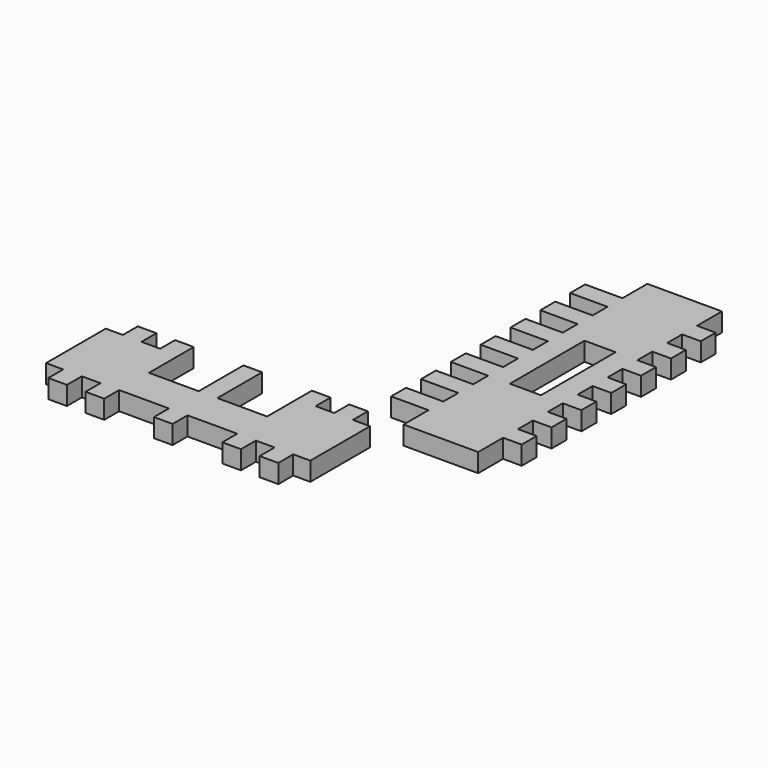
from build123d import *

# Parameters (mm, degrees)
F0_W     = 3
F0_H     = 3
F1_DEPTH = 3
F2_W     = 5
F2_H     = 15
F3_DEPTH = 25


# Not quite as in the source:
# - a feature names something its author has since deleted; it is built from what else it names


with BuildPart() as f1:
    # F0 (on Top) → F1 (new body)
    with BuildSketch(Plane.XY):
        Polygon((20.2673766234, -38.1281147589), (20.2673766234, -26.1281147589), (17.5173766234, -26.1281147589), (17.5173766234, -29.1281147589), (14.5173766234, -29.1281147589), (14.5173766234, -26.1281147589), (11.5173766234, -26.1281147589), (11.5173766234, -29.1281147589), (8.5173766234, -29.1281147589), (8.5173766234, -32.1281147589), (0.5173766234, -32.1281147589), (0.5173766234, -29.1281147589), (-2.4826233766, -29.1281147589), (-2.4826233766, -32.1281147589), (-10.4826233766, -32.1281147589), (-10.4826233766, -29.1281147589), (-13.4826233766, -29.1281147589), (-13.4826233766, -26.1281147589), (-16.4826233766, -26.1281147589), (-16.4826233766, -29.1281147589), (-19.4826233766, -29.1281147589), (-19.4826233766, -26.1281147589), (-22.2326233766, -26.1281147589), (-22.2326233766, -32.1281147589), (-22.2326233766, -38.1281147589), (-19.4826233766, -38.1281147589), (-19.4826233766, -35.1281147589), (-16.4826233766, -35.1281147589), (-16.4826233766, -38.1281147589), (-13.4826233766, -38.1281147589), (-13.4826233766, -35.1281147589), (-10.4826233766, -35.1281147589), (-10.4826233766, -38.1281147589), (-2.4826233766, -38.1281147589), (-2.4826233766, -35.1281147589), (0.5173766234, -35.1281147589), (0.5173766234, -38.1281147589), (8.5173766234, -38.1281147589), (8.5173766234, -35.1281147589), (11.5173766234, -35.1281147589), (11.5173766234, -38.1281147589), (14.5173766234, -38.1281147589), (14.5173766234, -35.1281147589), (17.5173766234, -35.1281147589), (17.5173766234, -38.1281147589), align=None)
        with Locations((16.0173766234, -27.6281147589)):
            Rectangle(F0_W, F0_H)
        with Locations((16.0173766234, -24.6281147589)):
            Rectangle(F0_W, F0_H)
        with Locations((16.0173766234, -39.6281147589)):
            Rectangle(F0_W, F0_H)
        with Locations((16.0173766234, -36.6281147589)):
            Rectangle(F0_W, F0_H)
        with Locations((10.0173766234, -27.6281147589)):
            Rectangle(F0_W, F0_H)
        with Locations((10.0173766234, -24.6281147589)):
            Rectangle(F0_W, F0_H)
        with Locations((10.0173766234, -39.6281147589)):
            Rectangle(F0_W, F0_H)
        with Locations((10.0173766234, -36.6281147589)):
            Rectangle(F0_W, F0_H)
        Polygon((0.5173766234, -27.6126158823), (0.5173766234, -26.1281147589), (-2.4826233766, -26.1281147589), (-2.4826233766, -29.1281147589), (0.5173766234, -29.1281147589), align=None)
        with Locations((-0.9826233766, -24.6281147589)):
            Rectangle(F0_W, F0_H)
        with Locations((-0.9826233766, -39.6281147589)):
            Rectangle(F0_W, F0_H)
        with Locations((-0.9826233766, -36.6281147589)):
            Rectangle(F0_W, F0_H)
        with Locations((-11.9826233766, -27.6281147589)):
            Rectangle(F0_W, F0_H)
        with Locations((-11.9826233766, -24.6281147589)):
            Rectangle(F0_W, F0_H)
        with Locations((-11.9826233766, -39.6281147589)):
            Rectangle(F0_W, F0_H)
        with Locations((-11.9826233766, -36.6281147589)):
            Rectangle(F0_W, F0_H)
        with Locations((-17.9826233766, -27.6281147589)):
            Rectangle(F0_W, F0_H)
        with Locations((-17.9826233766, -24.6281147589)):
            Rectangle(F0_W, F0_H)
        with Locations((-17.9826233766, -39.6281147589)):
            Rectangle(F0_W, F0_H)
        with Locations((-17.9826233766, -36.6281147589)):
            Rectangle(F0_W, F0_H)
    extrude(amount=F1_DEPTH)


with BuildPart() as f1b:
    # F0 (on Top) → F1, piece 2 (new body)
    with BuildSketch(Plane.XY):
        with Locations((18.7673766234, -16.6281147589)):
            Rectangle(F0_W, F0_H)
        with Locations((21.7673766234, -16.6281147589)):
            Rectangle(F0_W, F0_H)
        Polygon((23.2673766234, -15.1281147589), (23.2673766234, -18.1281147589), (23.2673766234, -23.1281147589), (35.2673766234, -23.1281147589), (35.2673766234, -18.1281147589), (35.2673766234, -15.1281147589), (35.2673766234, -12.1281147589), (35.2673766234, -9.1281147589), (35.2673766234, -6.1281147589), (35.2673766234, -3.1281147589), (35.2673766234, -0.1281147589), (35.2673766234, 2.8718852411), (35.2673766234, 5.8718852411), (35.2673766234, 8.8718852411), (35.2673766234, 11.8718852411), (35.2673766234, 14.8718852411), (35.2673766234, 17.8718852411), (35.2673766234, 20.8718852411), (35.2673766234, 25.8718852411), (29.2673766234, 25.8718852411), (23.2673766234, 25.8718852411), (23.2673766234, 20.8718852411), (23.2673766234, 17.8718852411), (23.2673766234, 14.8718852411), (23.2673766234, 11.8718852411), (23.2673766234, 8.8718852411), (23.2673766234, 5.8718852411), (23.2673766234, 2.8718852411), (23.2673766234, -0.1281147589), (23.2673766234, -3.1281147589), (23.2673766234, -6.1281147589), (23.2673766234, -9.1281147589), (23.2673766234, -12.1281147589), align=None)
        with Locations((18.7673766234, -10.6281147589)):
            Rectangle(F0_W, F0_H)
        with Locations((21.7673766234, -10.6281147589)):
            Rectangle(F0_W, F0_H)
        with Locations((18.7673766234, -4.6281147589)):
            Rectangle(F0_W, F0_H)
        with Locations((21.7673766234, -4.6281147589)):
            Rectangle(F0_W, F0_H)
        with Locations((36.7673766234, -16.6281147589)):
            Rectangle(F0_W, F0_H)
        with Locations((18.7673766234, 1.3718852411)):
            Rectangle(F0_W, F0_H)
        with Locations((21.7673766234, 1.3718852411)):
            Rectangle(F0_W, F0_H)
        with Locations((36.7673766234, -10.6281147589)):
            Rectangle(F0_W, F0_H)
        with Locations((18.7673766234, 7.3718852411)):
            Rectangle(F0_W, F0_H)
        with Locations((21.7673766234, 7.3718852411)):
            Rectangle(F0_W, F0_H)
        with Locations((36.7673766234, -4.6281147589)):
            Rectangle(F0_W, F0_H)
        with Locations((18.7673766234, 13.3718852411)):
            Rectangle(F0_W, F0_H)
        with Locations((21.7673766234, 13.3718852411)):
            Rectangle(F0_W, F0_H)
        with Locations((36.7673766234, 1.3718852411)):
            Rectangle(F0_W, F0_H)
        with Locations((18.7673766234, 19.3718852411)):
            Rectangle(F0_W, F0_H)
        with Locations((21.7673766234, 19.3718852411)):
            Rectangle(F0_W, F0_H)
        with Locations((36.7673766234, 7.3718852411)):
            Rectangle(F0_W, F0_H)
        with Locations((36.7673766234, 13.3718852411)):
            Rectangle(F0_W, F0_H)
        with Locations((36.7673766234, 19.3718852411)):
            Rectangle(F0_W, F0_H)
    extrude(amount=F1_DEPTH)

    # F2 (on Top) → F3 (cut)
    with BuildSketch(Plane.XY):
        with Locations((29.2673766234, 1.3718852411)):
            Rectangle(F2_W, F2_H)
    extrude(amount=F3_DEPTH, mode=Mode.SUBTRACT)


solid = Compound([f1.part, f1b.part])
